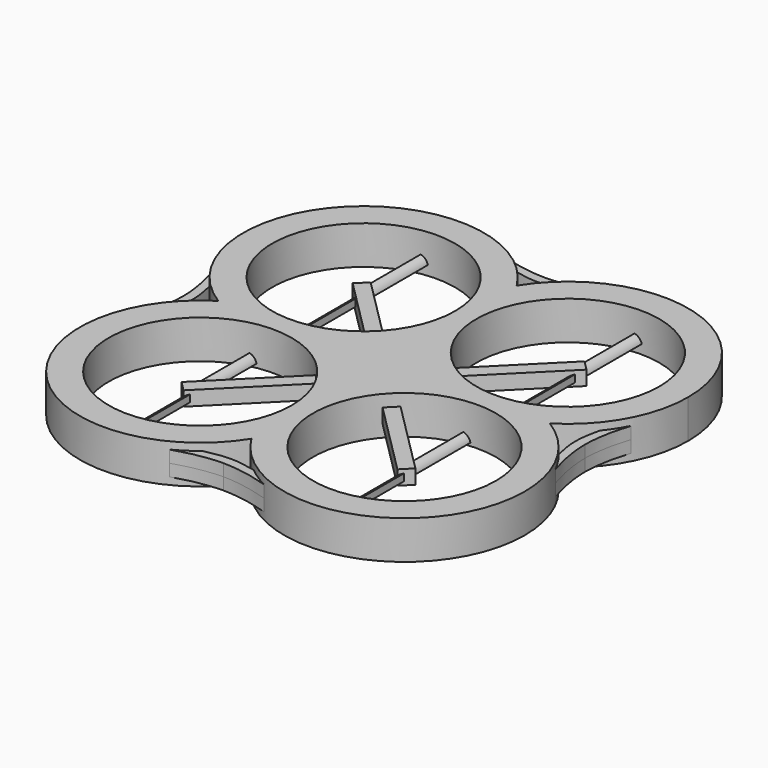
from build123d import *

# Parameters (mm, degrees)
F1_DEPTH      = 4
F2_R          = 19
F3_DEPTH      = 12.5
F5_DEPTH      = 2.5
F7_DEPTH      = 4
F9_DEPTH      = 1.5
F10_W         = 1.5
F10_H         = 32
F11_DEPTH     = 0.75
F12_T4_DEPTH  = 19.5164529043
F12_T9_DEPTH  = 19.5164529043
F12_T14_DEPTH = 22.8576067874
F12_T19_DEPTH = 18.0163776047
F12_T24_DEPTH = 19.5162583954
F12_T29_DEPTH = 19.5162583954
F12_T34_DEPTH = 24.3576067874
F12_T40_DEPTH = 19.5163776047
F12_T45_DEPTH = 22.8576067874
F12_T50_DEPTH = 18.0163776047
F12_T55_DEPTH = 19.5164529043
F12_T60_DEPTH = 19.5164529043
F12_T65_DEPTH = 24.3576067874
F12_T71_DEPTH = 19.5163776047
F12_T76_DEPTH = 19.5162583954
F12_T81_DEPTH = 19.5162583954


# Not quite as in the source:
# - a fillet or chamfer that OpenCascade refuses, or shapes differently, is made with other operations: its cross-section is extruded or revolved along the edge and cut away or added


with BuildPart() as f1:
    # F0 (on Top) → F1 (new body, symmetric)
    with BuildSketch(Plane.XY):
        with BuildLine():
            ThreePointArc((34.4419599909, 0), (43.0732001634, 9.0830532692), (46.2132034356, 21.2132034356))
            ThreePointArc((46.2132034356, 21.2132034356), (28.0932439191, 45.247866798), (0, 34.4419599909))
            ThreePointArc((0, 34.4419599909), (2.8214599268, 28.0932439191), (3.7867965644, 21.2132034356))
            ThreePointArc((3.7867965644, 21.2132034356), (2.8214599268, 14.3331629521), (0, 7.9844468803))
            ThreePointArc((0, 7.9844468803), (1.6409473913, 5.6592073787), (3.5355339059, 3.5355339059))
            ThreePointArc((3.5355339059, 3.5355339059), (5.6592073787, 1.6409473913), (7.9844468803, 0))
            ThreePointArc((7.9844468803, 0), (21.2132034356, 3.7867965644), (34.4419599909, 0))
        make_face()
        with BuildLine():
            ThreePointArc((3.7867965644, 21.2132034356), (2.8214599268, 28.0932439191), (0, 34.4419599909))
            ThreePointArc((0, 34.4419599909), (-3.7867965644, 21.2132034356), (0, 7.9844468803))
            ThreePointArc((0, 7.9844468803), (2.8214599268, 14.3331629521), (3.7867965644, 21.2132034356))
        make_face()
        with BuildLine():
            ThreePointArc((0, 7.9844468803), (-3.7867965644, 21.2132034356), (0, 34.4419599909))
            ThreePointArc((0, 34.4419599909), (-38.8908729653, 38.8908729653), (-34.4419599909, 0))
            ThreePointArc((-34.4419599909, 0), (-21.2132034356, 3.7867965644), (-7.9844468803, 0))
            ThreePointArc((-7.9844468803, 0), (-3.5355339059, 3.5355339059), (0, 7.9844468803))
        make_face()
        with BuildLine():
            ThreePointArc((46.2132034356, -21.2132034356), (43.0732001634, -9.0830532692), (34.4419599909, 0))
            ThreePointArc((34.4419599909, 0), (21.2132034356, -3.7867965644), (7.9844468803, 0))
            ThreePointArc((7.9844468803, 0), (3.5355339059, -3.5355339059), (0, -7.9844468803))
            ThreePointArc((0, -7.9844468803), (2.8214599268, -14.3331629521), (3.7867965644, -21.2132034356))
            ThreePointArc((3.7867965644, -21.2132034356), (2.8214599268, -28.0932439191), (0, -34.4419599909))
            ThreePointArc((0, -34.4419599909), (28.0932439191, -45.247866798), (46.2132034356, -21.2132034356))
        make_face()
        with BuildLine():
            ThreePointArc((7.9844468803, 0), (21.2132034356, -3.7867965644), (34.4419599909, 0))
            ThreePointArc((34.4419599909, 0), (21.2132034356, 3.7867965644), (7.9844468803, 0))
        make_face()
        with BuildLine():
            ThreePointArc((-7.9844468803, 0), (-21.2132034356, 3.7867965644), (-34.4419599909, 0))
            ThreePointArc((-34.4419599909, 0), (-21.2132034356, -3.7867965644), (-7.9844468803, 0))
        make_face()
        with BuildLine():
            ThreePointArc((-7.9844468803, 0), (-21.2132034356, -3.7867965644), (-34.4419599909, 0))
            ThreePointArc((-34.4419599909, 0), (-38.8908729653, -38.8908729653), (0, -34.4419599909))
            ThreePointArc((0, -34.4419599909), (-3.7867965644, -21.2132034356), (0, -7.9844468803))
            ThreePointArc((0, -7.9844468803), (-3.5355339059, -3.5355339059), (-7.9844468803, 0))
        make_face()
        with BuildLine():
            ThreePointArc((0, -7.9844468803), (-3.7867965644, -21.2132034356), (0, -34.4419599909))
            ThreePointArc((0, -34.4419599909), (2.8214599268, -28.0932439191), (3.7867965644, -21.2132034356))
            ThreePointArc((3.7867965644, -21.2132034356), (2.8214599268, -14.3331629521), (0, -7.9844468803))
        make_face()
    extrude(amount=F1_DEPTH, both=True)

    # F2 (on Top) → F3 (cut, symmetric)
    with BuildSketch(Plane.XY):
        with BuildLine():
            ThreePointArc((7.7781745931, 7.7781745931), (28.4841886505, 3.6594923179), (40.2132034356, 21.2132034356))
            ThreePointArc((40.2132034356, 21.2132034356), (13.9422182207, 38.7669145533), (7.7781745931, 7.7781745931))
        make_face()
        with Locations((-21.2132034356, 21.2132034356)):
            Circle(F2_R)
        with Locations((21.2132034356, -21.2132034356)):
            Circle(F2_R)
        with Locations((-21.2132034356, -21.2132034356)):
            Circle(F2_R)
    extrude(amount=F3_DEPTH, both=True, mode=Mode.SUBTRACT)

    # F4 (on Top) → F5 (join, symmetric)
    with BuildSketch(Plane.XY):
        with BuildLine():
            add(Edge.make_bspline(
                [(-10.8935860917, 43.6237454414), (-9.7174541894, 43.5485046), (-7.2638543693, 42.6049199754), (-3.4249107579, 41.9164425998), (-1.0230745432, 41.7217114309), (0, 41.7216904461)],
                knots=[0, 0, 0, 0, 0.3354940064, 0.6815384227, 1, 1, 1, 1], degree=3))
            Line((-10.8935860917, 43.6237454414), (-6.5460321493, 40.7336130738))
            add(Edge.make_bspline(
                [(-6.5460321493, 40.7336130738), (-5.4178979125, 40.5717682389), (-3.4146018114, 40.123397285), (-1.6052463196, 39.845453545), (-0.5105622517, 39.7925186696), (0, 39.7949367762)],
                knots=[0, 0, 0, 0, 0.4092670128, 0.7162515535, 1, 1, 1, 1], degree=3))
            add(Edge.make_bspline(
                [(6.5460321493, 40.7336130738), (5.4178979125, 40.5717682389), (3.4146018114, 40.123397285), (1.6052463196, 39.845453545), (0.5105622517, 39.7925186696), (0, 39.7949367762)],
                knots=[0, 0, 0, 0, 0.4092670128, 0.7162515535, 1, 1, 1, 1], degree=3))
            Line((6.5460321493, 40.7336130738), (10.8935860917, 43.6237454414))
            add(Edge.make_bspline(
                [(10.8935860917, 43.6237454414), (9.7174541894, 43.5485046), (7.2638543693, 42.6049199754), (3.4249107579, 41.9164425998), (1.0230745432, 41.7217114309), (0, 41.7216904461)],
                knots=[0, 0, 0, 0, 0.3354940064, 0.6815384227, 1, 1, 1, 1], degree=3))
        make_face()
        with BuildLine():
            Line((40.7336130738, -6.5460321493), (43.6237454414, -10.8935860917))
            add(Edge.make_bspline(
                [(43.6237454414, -10.8935860917), (43.5485046, -9.7174541894), (42.6049199754, -7.2638543693), (41.9164425998, -3.4249107579), (41.7217114309, -1.0230745432), (41.7216904461, 0)],
                knots=[0, 0, 0, 0, 0.3354940064, 0.6815384227, 1, 1, 1, 1], degree=3))
            add(Edge.make_bspline(
                [(43.6237454414, 10.8935860917), (43.5485046, 9.7174541894), (42.6049199754, 7.2638543693), (41.9164425998, 3.4249107579), (41.7217114309, 1.0230745432), (41.7216904461, 0)],
                knots=[0, 0, 0, 0, 0.3354940064, 0.6815384227, 1, 1, 1, 1], degree=3))
            Line((43.6237454414, 10.8935860917), (40.7336130738, 6.5460321493))
            add(Edge.make_bspline(
                [(40.7336130738, 6.5460321493), (40.5717682389, 5.4178979125), (40.123397285, 3.4146018114), (39.845453545, 1.6052463196), (39.7925186696, 0.5105622517), (39.7949367762, 0)],
                knots=[0, 0, 0, 0, 0.4092670128, 0.7162515535, 1, 1, 1, 1], degree=3))
            add(Edge.make_bspline(
                [(40.7336130738, -6.5460321493), (40.5717682389, -5.4178979125), (40.123397285, -3.4146018114), (39.845453545, -1.6052463196), (39.7925186696, -0.5105622517), (39.7949367762, 0)],
                knots=[0, 0, 0, 0, 0.4092670128, 0.7162515535, 1, 1, 1, 1], degree=3))
        make_face()
        with BuildLine():
            add(Edge.make_bspline(
                [(-43.6237454414, -10.8935860917), (-43.5485046, -9.7174541894), (-42.6049199754, -7.2638543693), (-41.9164425998, -3.4249107579), (-41.7217114309, -1.0230745432), (-41.7216904461, 0)],
                knots=[0, 0, 0, 0, 0.3354940064, 0.6815384227, 1, 1, 1, 1], degree=3))
            Line((-43.6237454414, -10.8935860917), (-40.7336130738, -6.5460321493))
            add(Edge.make_bspline(
                [(-40.7336130738, -6.5460321493), (-40.5717682389, -5.4178979125), (-40.123397285, -3.4146018114), (-39.845453545, -1.6052463196), (-39.7925186696, -0.5105622517), (-39.7949367762, 0)],
                knots=[0, 0, 0, 0, 0.4092670128, 0.7162515535, 1, 1, 1, 1], degree=3))
            add(Edge.make_bspline(
                [(-40.7336130738, 6.5460321493), (-40.5717682389, 5.4178979125), (-40.123397285, 3.4146018114), (-39.845453545, 1.6052463196), (-39.7925186696, 0.5105622517), (-39.7949367762, 0)],
                knots=[0, 0, 0, 0, 0.4092670128, 0.7162515535, 1, 1, 1, 1], degree=3))
            Line((-40.7336130738, 6.5460321493), (-43.6237454414, 10.8935860917))
            add(Edge.make_bspline(
                [(-43.6237454414, 10.8935860917), (-43.5485046, 9.7174541894), (-42.6049199754, 7.2638543693), (-41.9164425998, 3.4249107579), (-41.7217114309, 1.0230745432), (-41.7216904461, 0)],
                knots=[0, 0, 0, 0, 0.3354940064, 0.6815384227, 1, 1, 1, 1], degree=3))
        make_face()
        with BuildLine():
            add(Edge.make_bspline(
                [(10.8935860917, -43.6237454414), (9.7174541894, -43.5485046), (7.2638543693, -42.6049199754), (3.4249107579, -41.9164425998), (1.0230745432, -41.7217114309), (0, -41.7216904461)],
                knots=[0, 0, 0, 0, 0.3354940064, 0.6815384227, 1, 1, 1, 1], degree=3))
            Line((10.8935860917, -43.6237454414), (6.5460321493, -40.7336130738))
            add(Edge.make_bspline(
                [(6.5460321493, -40.7336130738), (5.4178979125, -40.5717682389), (3.4146018114, -40.123397285), (1.6052463196, -39.845453545), (0.5105622517, -39.7925186696), (0, -39.7949367762)],
                knots=[0, 0, 0, 0, 0.4092670128, 0.7162515535, 1, 1, 1, 1], degree=3))
            add(Edge.make_bspline(
                [(-6.5460321493, -40.7336130738), (-5.4178979125, -40.5717682389), (-3.4146018114, -40.123397285), (-1.6052463196, -39.845453545), (-0.5105622517, -39.7925186696), (0, -39.7949367762)],
                knots=[0, 0, 0, 0, 0.4092670128, 0.7162515535, 1, 1, 1, 1], degree=3))
            Line((-6.5460321493, -40.7336130738), (-10.8935860917, -43.6237454414))
            add(Edge.make_bspline(
                [(-10.8935860917, -43.6237454414), (-9.7174541894, -43.5485046), (-7.2638543693, -42.6049199754), (-3.4249107579, -41.9164425998), (-1.0230745432, -41.7217114309), (0, -41.7216904461)],
                knots=[0, 0, 0, 0, 0.3354940064, 0.6815384227, 1, 1, 1, 1], degree=3))
        make_face()
    extrude(amount=F5_DEPTH, both=True)

    # F6 (on Top) → F7 (join, symmetric)
    with BuildSketch(Plane.XY):
        with BuildLine():
            add(Edge.make_bspline(
                [(0, 21.6244887561), (1.5220498899, 21.2535466999), (2.8868712412, 14.0087190699), (6.0590090616, 9.019654728), (8.8693268252, 3.0184376664), (9.0880226344, 0)],
                knots=[0, 0, 0, 0, 0.3236785064, 0.637767206, 1, 1, 1, 1], degree=3))
            add(Edge.make_bspline(
                [(0, 21.6244887561), (-1.5220498899, 21.2535466999), (-2.8868712412, 14.0087190699), (-6.0590090616, 9.019654728), (-8.8693268252, 3.0184376664), (-9.0880226344, 0)],
                knots=[0, 0, 0, 0, 0.3236785064, 0.637767206, 1, 1, 1, 1], degree=3))
            add(Edge.make_bspline(
                [(0, -21.6244887561), (-1.5220498899, -21.2535466999), (-2.8868712412, -14.0087190699), (-6.0590090616, -9.019654728), (-8.8693268252, -3.0184376664), (-9.0880226344, 0)],
                knots=[0, 0, 0, 0, 0.3236785064, 0.637767206, 1, 1, 1, 1], degree=3))
            add(Edge.make_bspline(
                [(0, -21.6244887561), (1.5220498899, -21.2535466999), (2.8868712412, -14.0087190699), (6.0590090616, -9.019654728), (8.8693268252, -3.0184376664), (9.0880226344, 0)],
                knots=[0, 0, 0, 0, 0.3236785064, 0.637767206, 1, 1, 1, 1], degree=3))
        make_face()
    extrude(amount=F7_DEPTH, both=True)

    # F8 (on Top) → F9 (join, symmetric)
    with BuildSketch(Plane.XY):
        Polygon((-22.2132034356, 20.1382922529), (-2.0749111827, 0), (-22.2132034356, -20.1382922529), (-20.1382922529, -22.2132034356), (0, -2.0749111827), (20.1382922529, -22.2132034356), (22.2132034356, -20.1382922529), (2.0749111827, 0), (22.2132034356, 20.1382922529), (20.1382922529, 22.2132034356), (0, 2.0749111827), (-20.1382922529, 22.2132034356), align=None)
        Polygon((-22.2132034356, 22.2132034356), (-22.2132034356, 20.1382922529), (-20.1382922529, 22.2132034356), align=None)
        Polygon((-23.2132034356, 21.1382922529), (-22.2132034356, 20.1382922529), (-22.2132034356, 22.2132034356), align=None)
        Polygon((-22.2132034356, -22.2132034356), (-22.2132034356, -20.1382922529), (-23.2132034356, -21.1382922529), align=None)
        Polygon((-20.1382922529, -22.2132034356), (-22.2132034356, -20.1382922529), (-22.2132034356, -22.2132034356), align=None)
        Polygon((-23.2881146183, 21.2132034356), (-23.2132034356, 21.1382922529), (-22.2132034356, 22.2132034356), (-24.2881146183, 22.2132034356), align=None)
        Polygon((-22.2132034356, 22.2132034356), (-20.1382922529, 22.2132034356), (-21.2132034356, 23.2881146183), align=None)
        Polygon((-22.2132034356, 24.2881146183), (-22.2132034356, 22.2132034356), (-21.2132034356, 23.2881146183), align=None)
        Polygon((-24.2881146183, 22.2132034356), (-22.2132034356, 22.2132034356), (-22.2132034356, 24.2881146183), align=None)
        Polygon((-22.2132034356, -22.2132034356), (-23.2132034356, -21.1382922529), (-23.2881146183, -21.2132034356), (-24.2881146183, -22.2132034356), align=None)
        Polygon((-21.2132034356, -23.2881146183), (-20.1382922529, -22.2132034356), (-22.2132034356, -22.2132034356), align=None)
        Polygon((-22.2132034356, -24.2881146183), (-22.2132034356, -22.2132034356), (-24.2881146183, -22.2132034356), align=None)
        Polygon((-21.2132034356, -23.2881146183), (-22.2132034356, -22.2132034356), (-22.2132034356, -24.2881146183), align=None)
        Polygon((22.2132034356, 22.2132034356), (20.1382922529, 22.2132034356), (22.2132034356, 20.1382922529), align=None)
        Polygon((21.2132034356, 23.2881146183), (20.1382922529, 22.2132034356), (22.2132034356, 22.2132034356), align=None)
        Polygon((22.2132034356, -22.2132034356), (20.1382922529, -22.2132034356), (21.2132034356, -23.2881146183), align=None)
        Polygon((22.2132034356, -20.1382922529), (20.1382922529, -22.2132034356), (22.2132034356, -22.2132034356), align=None)
        Polygon((22.2132034356, 24.2881146183), (21.2132034356, 23.2881146183), (22.2132034356, 22.2132034356), align=None)
        Polygon((22.2132034356, 22.2132034356), (22.2132034356, 20.1382922529), (23.2132034356, 21.1382922529), align=None)
        Polygon((24.2881146183, 22.2132034356), (22.2132034356, 22.2132034356), (23.2132034356, 21.1382922529), (23.2881146183, 21.2132034356), align=None)
        Polygon((22.2132034356, 24.2881146183), (22.2132034356, 22.2132034356), (24.2881146183, 22.2132034356), align=None)
        Polygon((22.2132034356, -22.2132034356), (21.2132034356, -23.2881146183), (22.2132034356, -24.2881146183), align=None)
        Polygon((22.2132034356, -20.1382922529), (22.2132034356, -22.2132034356), (23.2132034356, -21.1382922529), align=None)
        Polygon((24.2881146183, -22.2132034356), (22.2132034356, -22.2132034356), (22.2132034356, -24.2881146183), align=None)
        Polygon((23.2132034356, -21.1382922529), (22.2132034356, -22.2132034356), (24.2881146183, -22.2132034356), (23.2881146183, -21.2132034356), align=None)
    extrude(amount=F9_DEPTH, both=True)

    # F10 (on Top) → F11 (join, symmetric)
    with BuildSketch(Plane.XY):
        with Locations((-22.2133006901, 22.2132410854)):
            Rectangle(F10_W, F10_H)
        with Locations((22.2133006901, 22.2132410854)):
            Rectangle(F10_W, F10_H)
        with Locations((-22.2133006901, -22.2132410854)):
            Rectangle(F10_W, F10_H)
        with Locations((22.2133006901, -22.2132410854)):
            Rectangle(F10_W, F10_H)
    extrude(amount=F11_DEPTH, both=True)

    # F12: fillet of radius 2 on 8 edges, made by hand


with BuildPart() as f12_tool2:
    # F12_s3 → F12_t4 (new body)
    with BuildSketch(Plane.XZ.offset(-18.6967881811)):
        with BuildLine():
            ThreePointArc((21.026809017, 0.75), (22.2515538883, 0.3311388301), (22.9633006901, -0.75))
            Line((22.9633006901, -0.75), (22.9633006901, 0.75))
            Line((22.9633006901, 0.75), (21.026809017, 0.75))
        make_face()
    extrude(amount=-F12_T4_DEPTH)

    split(bisect_by=Plane(origin=(23.250659027, 23.250659027, 0), x_dir=(0, 0, 1), z_dir=(0.7071067812, 0.7071067812, 0)), keep=Keep.TOP)


with BuildPart() as f1_1:
    add(f1.part)

    # F12_t1: cut F12_tool2
    add(f12_tool2.part, mode=Mode.SUBTRACT)


with BuildPart() as f12_tool7:
    # F12_s8 → F12_t9 (new body)
    with BuildSketch(Plane.XZ.offset(-18.6967881811)):
        with BuildLine():
            ThreePointArc((21.026809017, 0.75), (22.2515538883, 0.3311388301), (22.9633006901, -0.75))
            Line((22.9633006901, -0.75), (22.9633006901, 0.75))
            Line((22.9633006901, 0.75), (21.026809017, 0.75))
        make_face()
    extrude(amount=-F12_T9_DEPTH)

    split(bisect_by=Plane(origin=(-1.0374555914, 1.0374555914, 0), x_dir=(0, 0, 1), z_dir=(-0.7071067812, 0.7071067812, 0)), keep=Keep.TOP)


with BuildPart() as f1_2:
    add(f1_1.part)

    # F12_t6: cut F12_tool7
    add(f12_tool7.part, mode=Mode.SUBTRACT)


with BuildPart() as f12_tool12:
    # F12_s13 → F12_t14 (new body)
    with BuildSketch(Plane.XZ.offset(-24.2296186901)):
        with BuildLine():
            ThreePointArc((22.9633006901, 0.75), (21.88216186, 0.0382531983), (21.4633006901, -1.1864916731))
            Line((21.4633006901, -1.1864916731), (21.4633006901, 0.75))
            Line((21.4633006901, 0.75), (22.9633006901, 0.75))
        make_face()
    extrude(amount=F12_T14_DEPTH)

    split(bisect_by=Plane(origin=(23.250659027, 23.250659027, 0), x_dir=(0, 0, 1), z_dir=(0.7071067812, 0.7071067812, 0)), keep=Keep.TOP)


with BuildPart() as f1_3:
    add(f1_2.part)

    # F12_t11: cut F12_tool12
    add(f12_tool12.part, mode=Mode.SUBTRACT)


with BuildPart() as f12_tool17:
    # F12_s18 → F12_t19 (new body)
    with BuildSketch(Plane.XZ.offset(-24.2296186901)):
        with BuildLine():
            ThreePointArc((22.9633006901, 0.75), (21.88216186, 0.0382531983), (21.4633006901, -1.1864916731))
            Line((21.4633006901, -1.1864916731), (21.4633006901, 0.75))
            Line((21.4633006901, 0.75), (22.9633006901, 0.75))
        make_face()
    extrude(amount=F12_T19_DEPTH)

    split(bisect_by=Plane(origin=(1.0374555914, -1.0374555914, 0), x_dir=(0, 0, 1), z_dir=(0.7071067812, -0.7071067812, 0)), keep=Keep.TOP)


with BuildPart() as f1_4:
    add(f1_3.part)

    # F12_t16: cut F12_tool17
    add(f12_tool17.part, mode=Mode.SUBTRACT)


with BuildPart() as f12_tool22:
    # F12_s23 → F12_t24 (new body)
    with BuildSketch(Plane.XZ.offset(-18.69698269)):
        with BuildLine():
            ThreePointArc((-23.3997923632, 0.75), (-22.1750474918, 0.3311388301), (-21.4633006901, -0.75))
            Line((-21.4633006901, -0.75), (-21.4633006901, 0.75))
            Line((-21.4633006901, 0.75), (-23.3997923632, 0.75))
        make_face()
    extrude(amount=-F12_T24_DEPTH)

    split(bisect_by=Plane(origin=(1.0374555914, 1.0374555914, 0), x_dir=(0, 0, 1), z_dir=(0.7071067812, 0.7071067812, 0)), keep=Keep.TOP)


with BuildPart() as f1_5:
    add(f1_4.part)

    # F12_t21: cut F12_tool22
    add(f12_tool22.part, mode=Mode.SUBTRACT)


with BuildPart() as f12_tool27:
    # F12_s28 → F12_t29 (new body)
    with BuildSketch(Plane.XZ.offset(-18.69698269)):
        with BuildLine():
            ThreePointArc((-23.3997923632, 0.75), (-22.1750474918, 0.3311388301), (-21.4633006901, -0.75))
            Line((-21.4633006901, -0.75), (-21.4633006901, 0.75))
            Line((-21.4633006901, 0.75), (-23.3997923632, 0.75))
        make_face()
    extrude(amount=-F12_T29_DEPTH)

    split(bisect_by=Plane(origin=(-23.250659027, 23.250659027, 0), x_dir=(0, 0, 1), z_dir=(-0.7071067812, 0.7071067812, 0)), keep=Keep.TOP)


with BuildPart() as f1_6:
    add(f1_5.part)

    # F12_t26: cut F12_tool27
    add(f12_tool27.part, mode=Mode.SUBTRACT)


with BuildPart() as f12_tool32:
    # F12_s33 → F12_t34 (new body)
    with BuildSketch(Plane.XZ.offset(-25.7296186901)):
        with BuildLine():
            ThreePointArc((-21.4633006901, 0.75), (-22.5444395201, 0.0382531983), (-22.9633006901, -1.1864916731))
            Line((-22.9633006901, -1.1864916731), (-22.9633006901, 0.75))
            Line((-22.9633006901, 0.75), (-21.4633006901, 0.75))
        make_face()
    extrude(amount=F12_T34_DEPTH)

    split(bisect_by=Plane(origin=(1.0374555914, 1.0374555914, 0), x_dir=(0, 0, 1), z_dir=(0.7071067812, 0.7071067812, 0)), keep=Keep.TOP)

    split(bisect_by=Plane(origin=(-23.250659027, 23.250659027, 0), x_dir=(0, 0, 1), z_dir=(0.7071067812, -0.7071067812, 0)), keep=Keep.TOP)


with BuildPart() as f1_7:
    add(f1_6.part)

    # F12_t31: cut F12_tool32
    add(f12_tool32.part, mode=Mode.SUBTRACT)


with BuildPart() as f12_tool38:
    # F12_s39 → F12_t40 (new body)
    with BuildSketch(Plane.XZ.offset(-25.7296186901)):
        with BuildLine():
            ThreePointArc((-21.4633006901, 0.75), (-22.5444395201, 0.0382531983), (-22.9633006901, -1.1864916731))
            Line((-22.9633006901, -1.1864916731), (-22.9633006901, 0.75))
            Line((-22.9633006901, 0.75), (-21.4633006901, 0.75))
        make_face()
    extrude(amount=F12_T40_DEPTH)

    split(bisect_by=Plane(origin=(-1.0374555914, -1.0374555914, 0), x_dir=(0, 0, 1), z_dir=(-0.7071067812, -0.7071067812, 0)), keep=Keep.TOP)


with BuildPart() as f1_8:
    add(f1_7.part)

    # F12_t37: cut F12_tool38
    add(f12_tool38.part, mode=Mode.SUBTRACT)


with BuildPart() as f12_tool43:
    # F12_s44 → F12_t45 (new body)
    with BuildSketch(Plane.XZ.offset(24.2296186901)):
        with BuildLine():
            ThreePointArc((-22.9633006901, 0.75), (-21.88216186, 0.0382531983), (-21.4633006901, -1.1864916731))
            Line((-21.4633006901, -1.1864916731), (-21.4633006901, 0.75))
            Line((-21.4633006901, 0.75), (-22.9633006901, 0.75))
        make_face()
    extrude(amount=-F12_T45_DEPTH)

    split(bisect_by=Plane(origin=(-23.250659027, -23.250659027, 0), x_dir=(0, 0, 1), z_dir=(-0.7071067812, -0.7071067812, 0)), keep=Keep.TOP)


with BuildPart() as f1_9:
    add(f1_8.part)

    # F12_t42: cut F12_tool43
    add(f12_tool43.part, mode=Mode.SUBTRACT)


with BuildPart() as f12_tool48:
    # F12_s49 → F12_t50 (new body)
    with BuildSketch(Plane.XZ.offset(24.2296186901)):
        with BuildLine():
            ThreePointArc((-22.9633006901, 0.75), (-21.88216186, 0.0382531983), (-21.4633006901, -1.1864916731))
            Line((-21.4633006901, -1.1864916731), (-21.4633006901, 0.75))
            Line((-21.4633006901, 0.75), (-22.9633006901, 0.75))
        make_face()
    extrude(amount=-F12_T50_DEPTH)

    split(bisect_by=Plane(origin=(-1.0374555914, 1.0374555914, 0), x_dir=(0, 0, 1), z_dir=(-0.7071067812, 0.7071067812, 0)), keep=Keep.TOP)


with BuildPart() as f1_10:
    add(f1_9.part)

    # F12_t47: cut F12_tool48
    add(f12_tool48.part, mode=Mode.SUBTRACT)


with BuildPart() as f12_tool53:
    # F12_s54 → F12_t55 (new body)
    with BuildSketch(Plane.XZ.offset(18.6967881811)):
        with BuildLine():
            ThreePointArc((-21.026809017, 0.75), (-22.2515538883, 0.3311388301), (-22.9633006901, -0.75))
            Line((-22.9633006901, -0.75), (-22.9633006901, 0.75))
            Line((-22.9633006901, 0.75), (-21.026809017, 0.75))
        make_face()
    extrude(amount=F12_T55_DEPTH)

    split(bisect_by=Plane(origin=(-23.250659027, -23.250659027, 0), x_dir=(0, 0, 1), z_dir=(-0.7071067812, -0.7071067812, 0)), keep=Keep.TOP)


with BuildPart() as f1_11:
    add(f1_10.part)

    # F12_t52: cut F12_tool53
    add(f12_tool53.part, mode=Mode.SUBTRACT)


with BuildPart() as f12_tool58:
    # F12_s59 → F12_t60 (new body)
    with BuildSketch(Plane.XZ.offset(18.6967881811)):
        with BuildLine():
            ThreePointArc((-21.026809017, 0.75), (-22.2515538883, 0.3311388301), (-22.9633006901, -0.75))
            Line((-22.9633006901, -0.75), (-22.9633006901, 0.75))
            Line((-22.9633006901, 0.75), (-21.026809017, 0.75))
        make_face()
    extrude(amount=F12_T60_DEPTH)

    split(bisect_by=Plane(origin=(1.0374555914, -1.0374555914, 0), x_dir=(0, 0, 1), z_dir=(0.7071067812, -0.7071067812, 0)), keep=Keep.TOP)


with BuildPart() as f1_12:
    add(f1_11.part)

    # F12_t57: cut F12_tool58
    add(f12_tool58.part, mode=Mode.SUBTRACT)


with BuildPart() as f12_tool63:
    # F12_s64 → F12_t65 (new body)
    with BuildSketch(Plane.XZ.offset(25.7296186901)):
        with BuildLine():
            ThreePointArc((21.4633006901, 0.75), (22.5444395201, 0.0382531983), (22.9633006901, -1.1864916731))
            Line((22.9633006901, -1.1864916731), (22.9633006901, 0.75))
            Line((22.9633006901, 0.75), (21.4633006901, 0.75))
        make_face()
    extrude(amount=-F12_T65_DEPTH)

    split(bisect_by=Plane(origin=(-1.0374555914, -1.0374555914, 0), x_dir=(0, 0, 1), z_dir=(-0.7071067812, -0.7071067812, 0)), keep=Keep.TOP)

    split(bisect_by=Plane(origin=(23.250659027, -23.250659027, 0), x_dir=(0, 0, 1), z_dir=(-0.7071067812, 0.7071067812, 0)), keep=Keep.TOP)


with BuildPart() as f1_13:
    add(f1_12.part)

    # F12_t62: cut F12_tool63
    add(f12_tool63.part, mode=Mode.SUBTRACT)


with BuildPart() as f12_tool69:
    # F12_s70 → F12_t71 (new body)
    with BuildSketch(Plane.XZ.offset(25.7296186901)):
        with BuildLine():
            ThreePointArc((21.4633006901, 0.75), (22.5444395201, 0.0382531983), (22.9633006901, -1.1864916731))
            Line((22.9633006901, -1.1864916731), (22.9633006901, 0.75))
            Line((22.9633006901, 0.75), (21.4633006901, 0.75))
        make_face()
    extrude(amount=-F12_T71_DEPTH)

    split(bisect_by=Plane(origin=(1.0374555914, 1.0374555914, 0), x_dir=(0, 0, 1), z_dir=(0.7071067812, 0.7071067812, 0)), keep=Keep.TOP)


with BuildPart() as f1_14:
    add(f1_13.part)

    # F12_t68: cut F12_tool69
    add(f12_tool69.part, mode=Mode.SUBTRACT)


with BuildPart() as f12_tool74:
    # F12_s75 → F12_t76 (new body)
    with BuildSketch(Plane.XZ.offset(18.69698269)):
        with BuildLine():
            ThreePointArc((23.3997923632, 0.75), (22.1750474918, 0.3311388301), (21.4633006901, -0.75))
            Line((21.4633006901, -0.75), (21.4633006901, 0.75))
            Line((21.4633006901, 0.75), (23.3997923632, 0.75))
        make_face()
    extrude(amount=F12_T76_DEPTH)

    split(bisect_by=Plane(origin=(-1.0374555914, -1.0374555914, 0), x_dir=(0, 0, 1), z_dir=(-0.7071067812, -0.7071067812, 0)), keep=Keep.TOP)


with BuildPart() as f1_15:
    add(f1_14.part)

    # F12_t73: cut F12_tool74
    add(f12_tool74.part, mode=Mode.SUBTRACT)


with BuildPart() as f12_tool79:
    # F12_s80 → F12_t81 (new body)
    with BuildSketch(Plane.XZ.offset(18.69698269)):
        with BuildLine():
            ThreePointArc((23.3997923632, 0.75), (22.1750474918, 0.3311388301), (21.4633006901, -0.75))
            Line((21.4633006901, -0.75), (21.4633006901, 0.75))
            Line((21.4633006901, 0.75), (23.3997923632, 0.75))
        make_face()
    extrude(amount=F12_T81_DEPTH)

    split(bisect_by=Plane(origin=(23.250659027, -23.250659027, 0), x_dir=(0, 0, 1), z_dir=(0.7071067812, -0.7071067812, 0)), keep=Keep.TOP)


with BuildPart() as f1_16:
    add(f1_15.part)

    # F12_t78: cut F12_tool79
    add(f12_tool79.part, mode=Mode.SUBTRACT)


solid = f1_16.part
